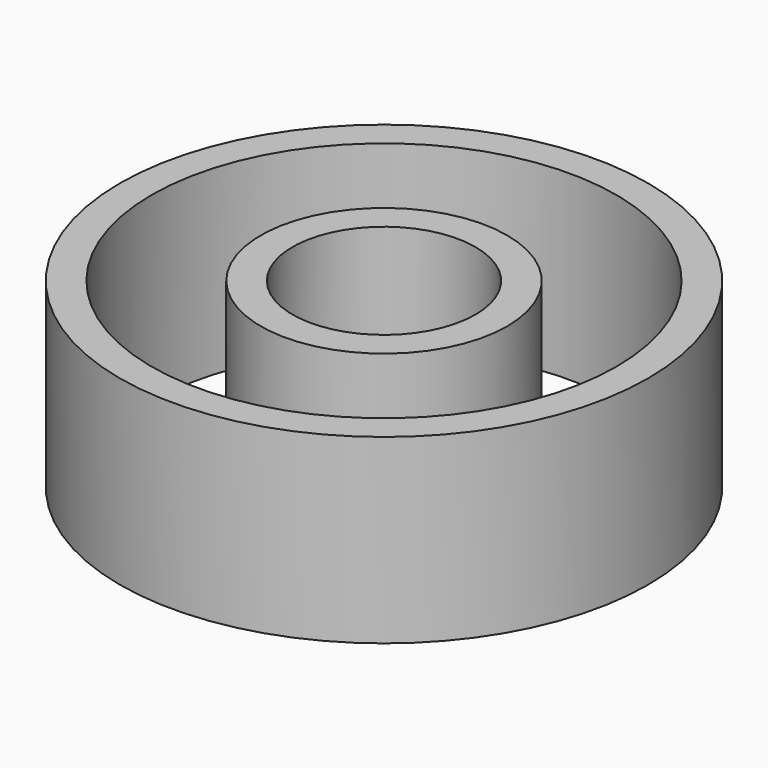
from build123d import *

# Parameters (mm, degrees)
F0_R     = 31.75
F0_R_2   = 27.94
F1_DEPTH = 21.844
F0_R_3   = 14.8082
F0_R_4   = 10.9982


# Not quite as in the source:
# - a feature names something its author has since deleted; it is built from what else it names


with BuildPart() as f1:
    # F0 (on Top) → F1 (new body)
    with BuildSketch(Plane.XY):
        with Locations((-65.6663700938, -42.8389012814)):
            Circle(F0_R)
        with Locations((-65.6663700938, -42.8389012814)):
            Circle(F0_R_2, mode=Mode.SUBTRACT)
    extrude(amount=F1_DEPTH)


with BuildPart() as f1b:
    # F0 (on Top) → F1, piece 2 (new body)
    with BuildSketch(Plane.XY):
        with Locations((-65.6663700938, -42.8389012814)):
            Circle(F0_R_3)
        with Locations((-65.6663700938, -42.8389012814)):
            Circle(F0_R_4, mode=Mode.SUBTRACT)
    extrude(amount=F1_DEPTH)


solid = Compound([f1.part, f1b.part])
